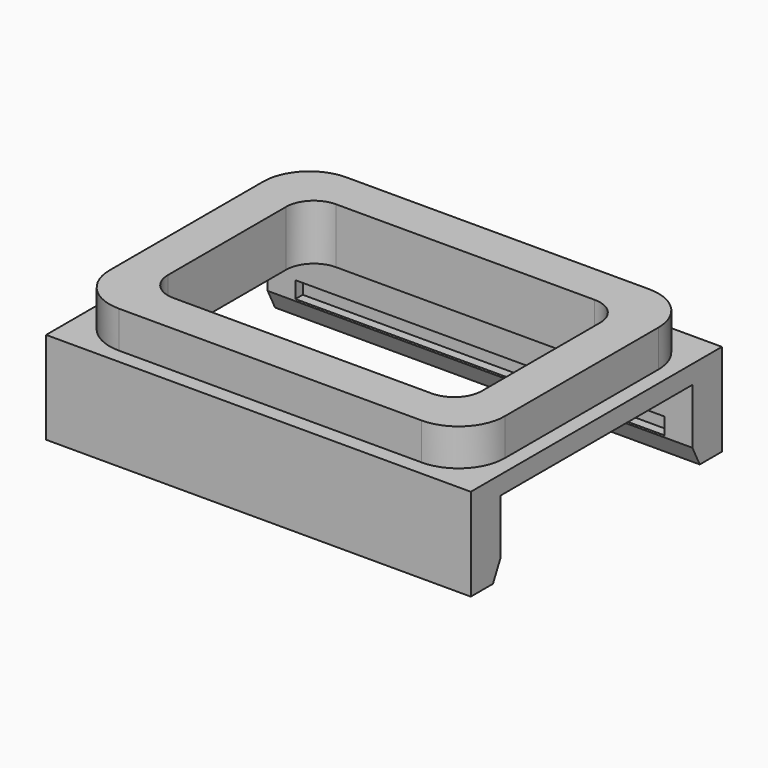
from build123d import *

# Parameters (mm, degrees)
F0_W         = 23
F0_H         = 17
F1_DEPTH     = 1
F2_DEPTH     = 3
F4_DEPTH     = 4
F5_DEPTH     = 2
F6_DEPTH     = 2
F7_W         = 1.5
F7_H         = 2
F8_DEPTH     = 4
F9_W         = 20
F9_H         = 1.1
F10_DEPTH    = 0.5
F11_W        = 20
F11_H        = 1.1
F12_DEPTH    = 0.5
F13_C1_SIZE2 = 1
F13_C1_SIZE  = 0.5
F13_C2_SIZE2 = 0.5
F13_C2_SIZE  = 1
F15_W        = 17
F15_H        = 11
F16_DEPTH    = 25
F17_R        = 1.5


# Not quite as in the source:
# - two fillets or chamfers of one size are made in one step


with BuildPart() as f1:
    # F0 (on Top) → F1 (new body)
    with BuildSketch(Plane.XY):
        Rectangle(F0_W, F0_H)
        with BuildLine():
            Line((-8.2, 7.7), (8.2, 7.7))
            ThreePointArc((8.2, 7.7), (9.967766953, 6.967766953), (10.7, 5.2))
            Line((10.7, 5.2), (10.7, -5.2))
            ThreePointArc((10.7, -5.2), (9.967766953, -6.967766953), (8.2, -7.7))
            Line((8.2, -7.7), (-8.2, -7.7))
            ThreePointArc((-8.2, -7.7), (-9.967766953, -6.967766953), (-10.7, -5.2))
            Line((-10.7, -5.2), (-10.7, 5.2))
            ThreePointArc((-10.7, 5.2), (-9.967766953, 6.967766953), (-8.2, 7.7))
        make_face(mode=Mode.SUBTRACT)
    extrude(amount=F1_DEPTH)

    # F0 (on Top) → F2 (join)
    with BuildSketch(Plane.XY):
        with BuildLine():
            ThreePointArc((10.7, 5.2), (9.967766953, 6.967766953), (8.2, 7.7))
            Line((8.2, 7.7), (-8.2, 7.7))
            ThreePointArc((-8.2, 7.7), (-9.967766953, 6.967766953), (-10.7, 5.2))
            Line((-10.7, 5.2), (-10.7, -5.2))
            ThreePointArc((-10.7, -5.2), (-9.967766953, -6.967766953), (-8.2, -7.7))
            Line((-8.2, -7.7), (8.2, -7.7))
            ThreePointArc((8.2, -7.7), (9.967766953, -6.967766953), (10.7, -5.2))
            Line((10.7, -5.2), (10.7, 5.2))
        make_face()
    extrude(amount=F2_DEPTH)

    # F3 (on face) → F4 (join)
    with BuildSketch(Plane.XY):
        with BuildLine():
            Line((10, -8.5), (10, -7))
            Line((10, -7), (9.9349351573, -7))
            ThreePointArc((9.9349351573, -7), (9.1354143467, -7.5184046239), (8.2, -7.7))
            Line((8.2, -7.7), (-8.2, -7.7))
            ThreePointArc((-8.2, -7.7), (-9.1354143467, -7.5184046239), (-9.9349351573, -7))
            Line((-9.9349351573, -7), (-10, -7))
            Line((-10, -7), (-10, -8.5))
            Line((-10, -8.5), (10, -8.5))
        make_face()
        with BuildLine():
            ThreePointArc((8.2, -7.7), (9.1354143467, -7.5184046239), (9.9349351573, -7))
            Line((9.9349351573, -7), (-9.9349351573, -7))
            ThreePointArc((-9.9349351573, -7), (-9.1354143467, -7.5184046239), (-8.2, -7.7))
            Line((-8.2, -7.7), (8.2, -7.7))
        make_face()
        with BuildLine():
            Line((9.9349351573, 7), (10, 7))
            Line((10, 7), (10, 8.5))
            Line((10, 8.5), (-10, 8.5))
            Line((-10, 8.5), (-10, 7))
            Line((-10, 7), (-9.9349351573, 7))
            ThreePointArc((-9.9349351573, 7), (-9.1354143467, 7.5184046239), (-8.2, 7.7))
            Line((-8.2, 7.7), (8.2, 7.7))
            ThreePointArc((8.2, 7.7), (9.1354143467, 7.5184046239), (9.9349351573, 7))
        make_face()
        with BuildLine():
            Line((-9.9349351573, 7), (9.9349351573, 7))
            ThreePointArc((9.9349351573, 7), (9.1354143467, 7.5184046239), (8.2, 7.7))
            Line((8.2, 7.7), (-8.2, 7.7))
            ThreePointArc((-8.2, 7.7), (-9.1354143467, 7.5184046239), (-9.9349351573, 7))
        make_face()
    extrude(amount=-F4_DEPTH)

    # F3 (on face) → F5 (join)
    with BuildSketch(Plane.XY):
        with BuildLine():
            Line((-9.9349351573, -7), (9.9349351573, -7))
            ThreePointArc((9.9349351573, -7), (9.967766953, -6.967766953), (10, -6.9349351573))
            Line((10, -6.9349351573), (10, -6.5))
            Line((10, -6.5), (-10, -6.5))
            Line((-10, -6.5), (-10, -6.9349351573))
            ThreePointArc((-10, -6.9349351573), (-9.967766953, -6.967766953), (-9.9349351573, -7))
        make_face()
        with BuildLine():
            Line((10, 6.5), (10, 6.9349351573))
            ThreePointArc((10, 6.9349351573), (9.967766953, 6.967766953), (9.9349351573, 7))
            Line((9.9349351573, 7), (-9.9349351573, 7))
            ThreePointArc((-9.9349351573, 7), (-9.967766953, 6.967766953), (-10, 6.9349351573))
            Line((-10, 6.9349351573), (-10, 6.5))
            Line((-10, 6.5), (10, 6.5))
        make_face()
    extrude(amount=-F5_DEPTH)

    # F3 (on face) → F6 (join)
    with BuildSketch(Plane.XY):
        with BuildLine():
            Line((9.9349351573, -7), (10, -7))
            Line((10, -7), (10, -6.9349351573))
            ThreePointArc((10, -6.9349351573), (9.967766953, -6.967766953), (9.9349351573, -7))
        make_face()
        with BuildLine():
            Line((-10, -7), (-9.9349351573, -7))
            ThreePointArc((-9.9349351573, -7), (-9.967766953, -6.967766953), (-10, -6.9349351573))
            Line((-10, -6.9349351573), (-10, -7))
        make_face()
        with BuildLine():
            ThreePointArc((9.9349351573, 7), (9.967766953, 6.967766953), (10, 6.9349351573))
            Line((10, 6.9349351573), (10, 7))
            Line((10, 7), (9.9349351573, 7))
        make_face()
        with BuildLine():
            Line((-10, 7), (-10, 6.9349351573))
            ThreePointArc((-10, 6.9349351573), (-9.967766953, 6.967766953), (-9.9349351573, 7))
            Line((-9.9349351573, 7), (-10, 7))
        make_face()
    extrude(amount=-F6_DEPTH)

    # F7 (on face) → F8 (join)
    with BuildSketch(Plane(origin=(0, 0, 0), x_dir=(1, 0, 0), z_dir=(0, 0, -1))):
        with Locations((10.75, 7.5)):
            Rectangle(F7_W, F7_H)
        with Locations((-10.75, 7.5)):
            Rectangle(F7_W, F7_H)
        with Locations((-10.75, -7.5)):
            Rectangle(F7_W, F7_H)
        with Locations((10.75, -7.5)):
            Rectangle(F7_W, F7_H)
    extrude(amount=F8_DEPTH)

    # F9 (on face) → F10 (join)
    with BuildSketch(Plane(origin=(0, -7, 0), x_dir=(-1, 0, 0), z_dir=(0, 1, 0))):
        with Locations((0, -3.45)):
            Rectangle(F9_W, F9_H)
    extrude(amount=F10_DEPTH)

    # F11 (on face) → F12 (join)
    with BuildSketch(Plane.XZ.offset(-7)):
        with Locations((0, -3.45)):
            Rectangle(F11_W, F11_H)
    extrude(amount=F12_DEPTH)

    # F13: chamfer of 0.5 x 1 on 2 edges, made by hand

    # F13_c1
    f13_c1_edges = [f1.edges().sort_by_distance(p)[0] for p in [
        (0, -6.5, -4),
    ]]
    f13_c1_side = f1.faces().sort_by_distance((0, -6.51, -4))[0]
    chamfer(f13_c1_edges, length=F13_C1_SIZE, length2=F13_C1_SIZE2, reference=f13_c1_side)

    # F13_c2
    f13_c2_edges = [f1.edges().sort_by_distance(p)[0] for p in [
        (0, 6.5, -4),
    ]]
    f13_c2_side = f1.faces().sort_by_distance((0, 6.5, -3.99))[0]
    chamfer(f13_c2_edges, length=F13_C2_SIZE, length2=F13_C2_SIZE2, reference=f13_c2_side)

    # F15 (on face) → F16 (cut)
    with BuildSketch(Plane.XY.offset(3)):
        Rectangle(F15_W, F15_H)
    extrude(amount=-F16_DEPTH, mode=Mode.SUBTRACT)

    # F17
    f17_edges = [f1.edges().sort_by_distance(p)[0] for p in [
        (-8.5, -5.5, 1.5),
        (-8.5, 5.5, 1.5),
        (8.5, 5.5, 1.5),
        (8.5, -5.5, 1.5),
    ]]
    fillet(f17_edges, radius=F17_R)


solid = f1.part
